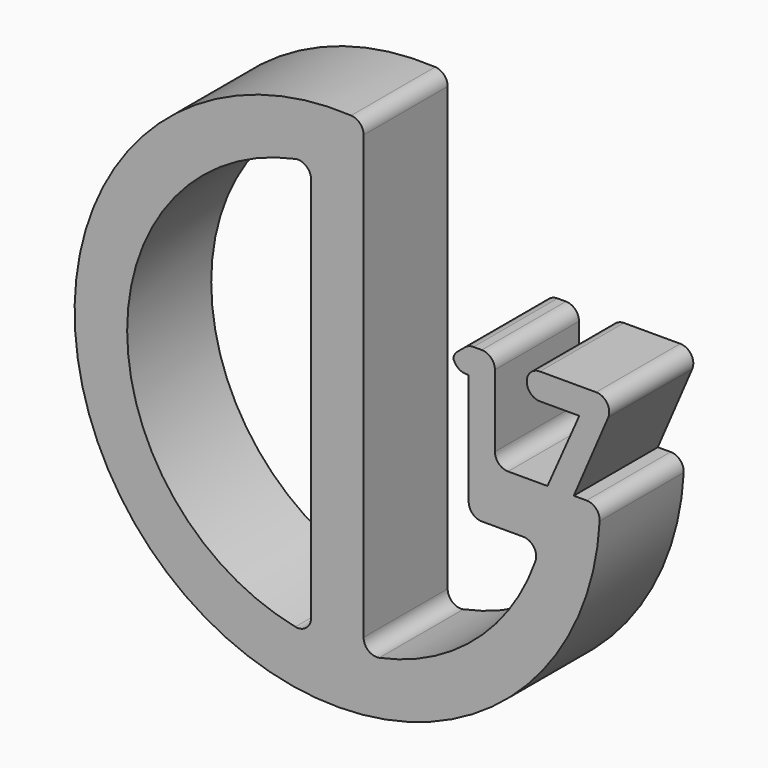
from build123d import *

# Parameters (mm, degrees)
F1_DEPTH     = 20
F2_T1_DEPTH  = 20
F2_T3_DEPTH  = 31.8767610709
F2_T5_DEPTH  = 38.9813299321
F2_T7_DEPTH  = 32.5
F2_T9_DEPTH  = 33.1624563251
F2_T11_DEPTH = 24.5256241898
F2_T13_DEPTH = 25.8546868248


# Not quite as in the source:
# - a fillet or chamfer that OpenCascade refuses, or shapes differently, is made with other operations: its cross-section is extruded or revolved along the edge and cut away or added


with BuildPart() as f1:
    # F0 (on Front) → F1 (new body)
    with BuildSketch(Plane.XZ):
        with BuildLine():
            Line((5, -39.686269666), (5, 0))
            Line((5, 0), (5, 49.7493718553))
            ThreePointArc((5, 49.7493718553), (-37.0809924355, -33.5410196625), (50, 0))
            Line((50, 0), (45, 0))
            Line((45, 0), (53.0514801827, 18.7251443562))
            Line((53.0514801827, 18.7251443562), (36.0514801827, 18.7251443562))
            Line((36.0514801827, 18.7251443562), (36.0514801827, 13.7251443562))
            Line((36.0514801827, 13.7251443562), (46.0514801827, 13.7251443562))
            Line((46.0514801827, 13.7251443562), (40, 0))
            Line((40, 0), (30, 0))
            Line((30, 0), (30, 18.7251443562))
            Line((30, 18.7251443562), (25, 18.7251443562))
            Line((25, 18.7251443562), (22, 16.2251443562))
            Line((22, 16.2251443562), (22, 13.7251443562))
            Line((22, 13.7251443562), (25, 13.7251443562))
            Line((25, 13.7251443562), (25, 0))
            Line((25, 0), (25, -10))
            Line((25, -10), (38.7298334621, -10))
            ThreePointArc((38.7298334621, -10), (26.4271306677, -30.0267674696), (5, -39.686269666))
        make_face()
        with BuildLine():
            Line((-5, 39.686269666), (-5, 0))
            Line((-5, 0), (-5, -39.686269666))
            ThreePointArc((-5, -39.686269666), (-40, 0), (-5, 39.686269666))
        make_face(mode=Mode.SUBTRACT)
    extrude(amount=F1_DEPTH)

    # F2: fillet of radius 2.5 on 15 edges, made by hand

    # F2_s2 → F2_t1 (join)
    with BuildSketch(Plane.XZ):
        with BuildLine():
            ThreePointArc((30, 2.5), (30.732233047, 0.732233047), (32.5, 0))
            Line((32.5, 0), (30, 0))
            Line((30, 0), (30, 2.5))
        make_face()
        with BuildLine():
            ThreePointArc((35.3553390593, -10), (37.3965805116, -11.056624327), (37.7123616633, -13.3333333333))
            ThreePointArc((37.7123616633, -13.3333333333), (38.2574185835, -11.677753351), (38.7298334621, -10))
            Line((38.7298334621, -10), (35.3553390593, -10))
        make_face()
        with BuildLine():
            ThreePointArc((-5, 36.7423461417), (-5.9188611699, 38.6788378149), (-8, 39.1918358845))
            ThreePointArc((-8, 39.1918358845), (-6.5046995466, 39.4675674929), (-5, 39.686269666))
            Line((-5, 39.686269666), (-5, 36.7423461417))
        make_face()
        with BuildLine():
            ThreePointArc((-5, -36.7423461417), (-5.9188611699, -38.6788378149), (-8, -39.1918358845))
            ThreePointArc((-8, -39.1918358845), (-6.5046995466, -39.4675674929), (-5, -39.686269666))
            Line((-5, -39.686269666), (-5, -36.7423461417))
        make_face()
        with BuildLine():
            ThreePointArc((5, -36.7423461417), (5.9188611699, -38.6788378149), (8, -39.1918358845))
            ThreePointArc((8, -39.1918358845), (6.5046995466, -39.4675674929), (5, -39.686269666))
            Line((5, -39.686269666), (5, -36.7423461417))
        make_face()
    extrude(amount=F2_T1_DEPTH)

    # F2_s4 → F2_t3 (cut)
    with BuildSketch(Plane.XZ.offset(-5.9383805354)):
        with BuildLine():
            ThreePointArc((5, 47.4341649025), (4.3136906253, 49.1547829066), (2.6315789474, 49.9306998974))
            ThreePointArc((2.6315789474, 49.9306998974), (3.8168664205, 49.8541024463), (5, 49.7493718553))
            Line((5, 49.7493718553), (5, 47.4341649025))
        make_face()
    extrude(amount=F2_T3_DEPTH, mode=Mode.SUBTRACT)

    # F2_s6 → F2_t5 (cut)
    with BuildSketch(Plane.XZ.offset(-9.490664966)):
        with BuildLine():
            ThreePointArc((51.5519019376, 15.2376093346), (51.3431363158, 17.6001284372), (49.2552141963, 18.7251443562))
            Line((49.2552141963, 18.7251443562), (53.0514801827, 18.7251443562))
            Line((53.0514801827, 18.7251443562), (51.5519019376, 15.2376093346))
        make_face()
    extrude(amount=F2_T5_DEPTH, mode=Mode.SUBTRACT)

    # F2_s8 → F2_t7 (cut)
    with BuildSketch(Plane.XZ.offset(-6.25)):
        with BuildLine():
            ThreePointArc((30, 16.2251443562), (29.267766953, 17.9929113092), (27.5, 18.7251443562))
            Line((27.5, 18.7251443562), (30, 18.7251443562))
            Line((30, 18.7251443562), (30, 16.2251443562))
        make_face()
        with BuildLine():
            ThreePointArc((22, 16.2251443562), (22.732233047, 14.4573774032), (24.5, 13.7251443562))
            Line((24.5, 13.7251443562), (22, 13.7251443562))
            Line((22, 13.7251443562), (22, 16.2251443562))
        make_face()
        with BuildLine():
            ThreePointArc((25, -7.5), (25.732233047, -9.267766953), (27.5, -10))
            Line((27.5, -10), (25, -10))
            Line((25, -10), (25, -7.5))
        make_face()
        with BuildLine():
            ThreePointArc((38.5514801827, 18.7251443562), (36.7837132297, 17.9929113092), (36.0514801827, 16.2251443562))
            Line((36.0514801827, 16.2251443562), (36.0514801827, 18.7251443562))
            Line((36.0514801827, 18.7251443562), (38.5514801827, 18.7251443562))
        make_face()
        with BuildLine():
            ThreePointArc((36.0514801827, 16.2251443562), (36.7837132297, 14.4573774032), (38.5514801827, 13.7251443562))
            Line((38.5514801827, 13.7251443562), (36.0514801827, 13.7251443562))
            Line((36.0514801827, 13.7251443562), (36.0514801827, 16.2251443562))
        make_face()
    extrude(amount=F2_T7_DEPTH, mode=Mode.SUBTRACT)

    # F2_s10 → F2_t9 (cut)
    with BuildSketch(Plane.XZ.offset(-6.5812281626)):
        with BuildLine():
            ThreePointArc((49.9306998974, -2.6315789474), (49.2478555278, -0.779381996), (47.4341649025, 0))
            Line((47.4341649025, 0), (50, 0))
            ThreePointArc((50, 0), (49.9826719717, -1.3162456325), (49.9306998974, -2.6315789474))
        make_face()
    extrude(amount=F2_T9_DEPTH, mode=Mode.SUBTRACT)

    # F2_s12 → F2_t11 (cut)
    with BuildSketch(Plane.XZ.offset(-2.2628120949)):
        with BuildLine():
            ThreePointArc((25.905124838, 18.7251443562), (25.0540616786, 18.5758233004), (24.3046638388, 18.1456975552))
            Line((24.3046638388, 18.1456975552), (25, 18.7251443562))
            Line((25, 18.7251443562), (25.905124838, 18.7251443562))
        make_face()
    extrude(amount=F2_T11_DEPTH, mode=Mode.SUBTRACT)

    # F2_s14 → F2_t13 (cut)
    with BuildSketch(Plane.XZ.offset(-2.9273434124)):
        with BuildLine():
            ThreePointArc((22.8995390008, 16.9747601902), (22.2360264469, 16.1145954819), (22, 15.0542069912))
            Line((22, 15.0542069912), (22, 16.2251443562))
            Line((22, 16.2251443562), (22.8995390008, 16.9747601902))
        make_face()
    extrude(amount=F2_T13_DEPTH, mode=Mode.SUBTRACT)


solid = f1.part
